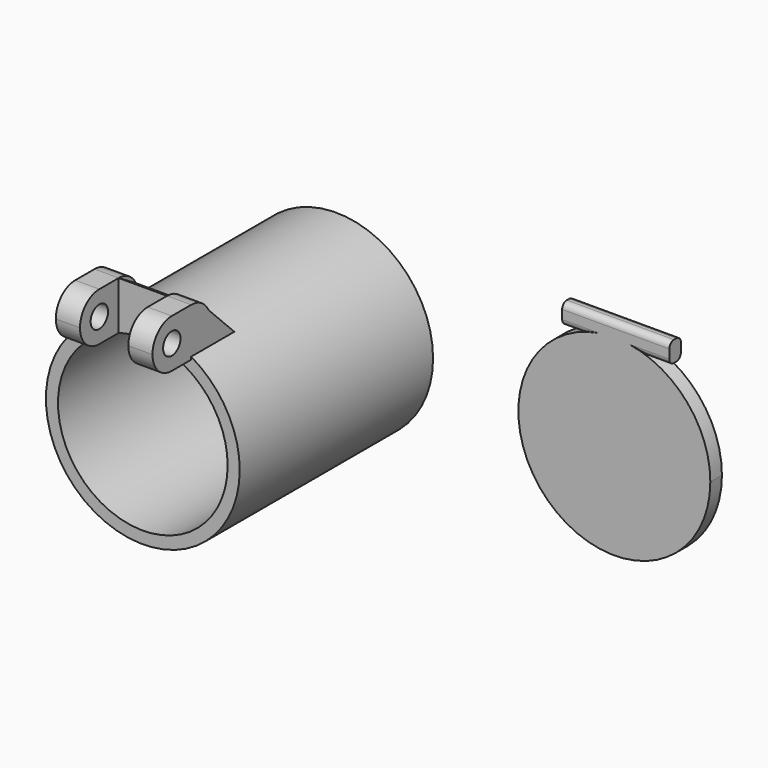
from build123d import *

# Parameters (mm, degrees)
F0_R      = 20.0498878018
F1_DEPTH  = 50
F2_T      = -2.5
F4_W      = 5
F4_H      = 10
F5_DEPTH  = 15
F6_R      = 4.99999
F8_D      = 4.5
F10_DEPTH = 3
F11_R     = 1.2
F13_DEPTH = 20


# Not quite as in the source:
# - a fillet or chamfer is up to 0.001 mm smaller than in the source, because OpenCascade refuses the exact size


with BuildPart() as f1:
    # F0 (on Front) → F1 (new body)
    with BuildSketch(Plane.XZ):
        with Locations((-20.4345174134, 1.8313954351)):
            Circle(F0_R)
    extrude(amount=F1_DEPTH)

    # F2
    f2_openings = [f1.faces().sort_by_distance(p)[0] for p in [
        (-20.434517, -50, 1.831395),
    ]]
    offset(amount=F2_T, openings=f2_openings)

    # F4 (on offset) → F5 (join)
    with BuildSketch(Plane.XZ.offset(45)):
        with Locations((-27.9345174134, 23.653956532)):
            Rectangle(F4_W, F4_H)
        with Locations((-12.9345174134, 23.653956532)):
            Rectangle(F4_W, F4_H)
    extrude(amount=F5_DEPTH)

    # F6 (radius 5 in the source; OpenCascade refuses exactly that, so slightly less here)
    f6_edges = [f1.edges().sort_by_distance(p)[0] for p in [
        (-12.934517, -45, 28.653957),
        (-27.934517, -45, 28.653957),
        (-27.934517, -60, 18.653957),
        (-12.934517, -60, 18.653957),
        (-12.934517, -60, 28.653957),
        (-27.934517, -60, 28.653957),
    ]]
    fillet(f6_edges, radius=F6_R)

    # F8 (through all)
    with Locations(Plane(origin=(-30.4345174134, 0, 0), x_dir=(0, -1, 0), z_dir=(-1, 0, 0))):
        with Locations((55, 23.653956532)):
            Hole(F8_D / 2)

    # F12 (on face) → F13 (join, through all)
    with BuildSketch(Plane(origin=(-30.4345174134, 0, 0), x_dir=(0, -1, 0), z_dir=(-1, 0, 0))):
        Polygon((38.8332865942, 19.2094851134), (45, 19.2094851134), (45.5421266796, 25.9183251988), align=None)
        Polygon((45.5421266796, 25.9183251988), (45, 19.2094851134), (50, 19.2094851134), (50, 28.653956532), align=None)
    extrude(amount=-F13_DEPTH)


with BuildPart() as f10:
    # F9 (on Front) → F10 (new body)
    with BuildSketch(Plane.XZ):
        with BuildLine():
            ThreePointArc((32.0807376184, 18.4103436768), (39.519585669, 19.8564149488), (46.9584337196, 18.4103436768))
            Line((46.9584337196, 18.4103436768), (50.8935190737, 18.4103436768))
            Line((50.8935190737, 18.4103436768), (50.8935190737, 22.6514711976))
            Line((50.8935190737, 22.6514711976), (28.72399427, 22.6514711976))
            Line((28.72399427, 22.6514711976), (28.72399427, 18.4103436768))
            Line((28.72399427, 18.4103436768), (32.0807376184, 18.4103436768))
        make_face()
        with BuildLine():
            ThreePointArc((32.0807376184, 18.4103436768), (28.4162447082, -16.4618660584), (59.3760006178, 0))
            ThreePointArc((59.3760006178, 0), (55.9814517275, 11.1033409608), (46.9584337196, 18.4103436768))
            Line((46.9584337196, 18.4103436768), (32.0807376184, 18.4103436768))
        make_face()
        with BuildLine():
            Line((32.0807376184, 18.4103436768), (46.9584337196, 18.4103436768))
            ThreePointArc((46.9584337196, 18.4103436768), (39.519585669, 19.8564149488), (32.0807376184, 18.4103436768))
        make_face()
    extrude(amount=F10_DEPTH)

    # F11
    f11_edges = [f10.edges().sort_by_distance(p)[0] for p in [
        (39.808757, 0, 22.651471),
        (39.808757, -3, 22.651471),
        (30.402366, 0, 18.410344),
        (48.925976, 0, 18.410344),
        (48.925976, -3, 18.410344),
        (30.402366, -3, 18.410344),
    ]]
    fillet(f11_edges, radius=F11_R)


solid = Compound([f1.part, f10.part])
